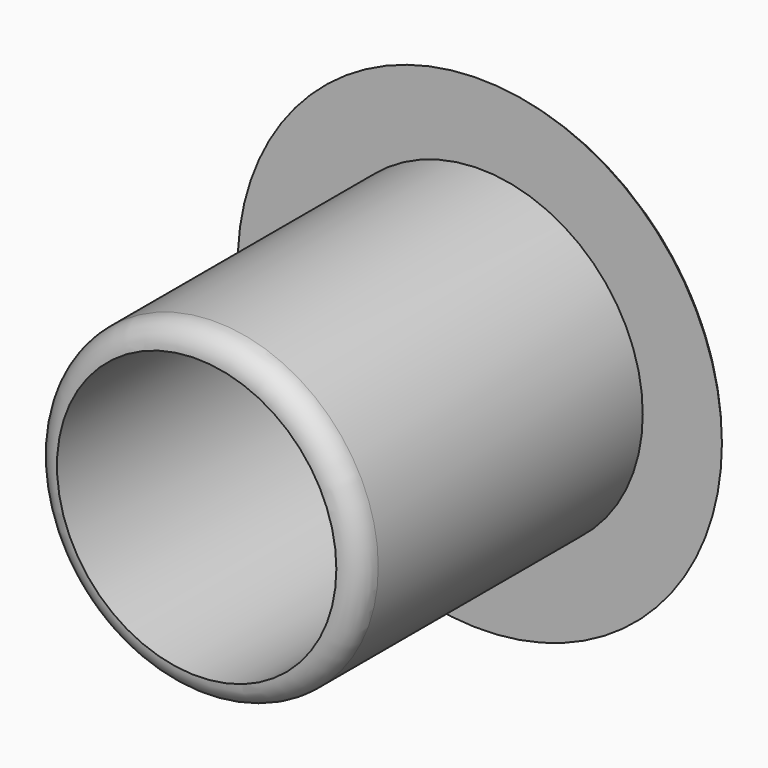
from build123d import *

# Parameters (mm, degrees)
F0_R     = 1.75
F0_R_2   = 1.5
F1_DEPTH = 4
F2_R     = 2.6
F2_R_2   = 1.75
F3_DEPTH = 0.2
F4_R     = 0.24999


# Not quite as in the source:
# - a fillet or chamfer that OpenCascade refuses, or shapes differently, is made with other operations: its cross-section is extruded or revolved along the edge and cut away or added
# - a fillet or chamfer is up to 0.001 mm smaller than in the source, because OpenCascade refuses the exact size


with BuildPart() as f1:
    # F0 (on Front) → F1 (new body)
    with BuildSketch(Plane.XZ):
        Circle(F0_R)
        Circle(F0_R_2, mode=Mode.SUBTRACT)
    extrude(amount=F1_DEPTH)

    # F2 (on Front) → F3 (join)
    with BuildSketch(Plane.XZ):
        Circle(F2_R)
        Circle(F2_R_2, mode=Mode.SUBTRACT)
    extrude(amount=F3_DEPTH)

    # F4 (radius 0.25 in the source; OpenCascade refuses exactly that, so slightly less here)
    f4_edges = [f1.edges().sort_by_distance(p)[0] for p in [
        (-1.75, -4, 0),
    ]]
    fillet(f4_edges, radius=F4_R)

    # F5: fillet of radius 0.5 on 2 edges, made by hand

    # F5_s1 → F5_t2 (revolve, cut)
    with BuildSketch(Plane.XY):
        with BuildLine():
            ThreePointArc((2.6, -0.2), (2.4236067977, -0.0527864045), (2.2, 0))
            Line((2.2, 0), (2.6, 0))
            Line((2.6, 0), (2.6, -0.2))
        make_face()
    revolve(axis=Axis((0, 0, 0), (0, -1, 0)), mode=Mode.SUBTRACT)

    # F5_s3 → F5_t4 (revolve, cut)
    with BuildSketch(Plane.XY):
        with BuildLine():
            ThreePointArc((1.5, -0.5), (1.6464466094, -0.1464466094), (2, 0))
            Line((2, 0), (1.5, 0))
            Line((1.5, 0), (1.5, -0.5))
        make_face()
    revolve(axis=Axis((0, 0, 0), (0, -1, 0)), mode=Mode.SUBTRACT)


solid = f1.part
